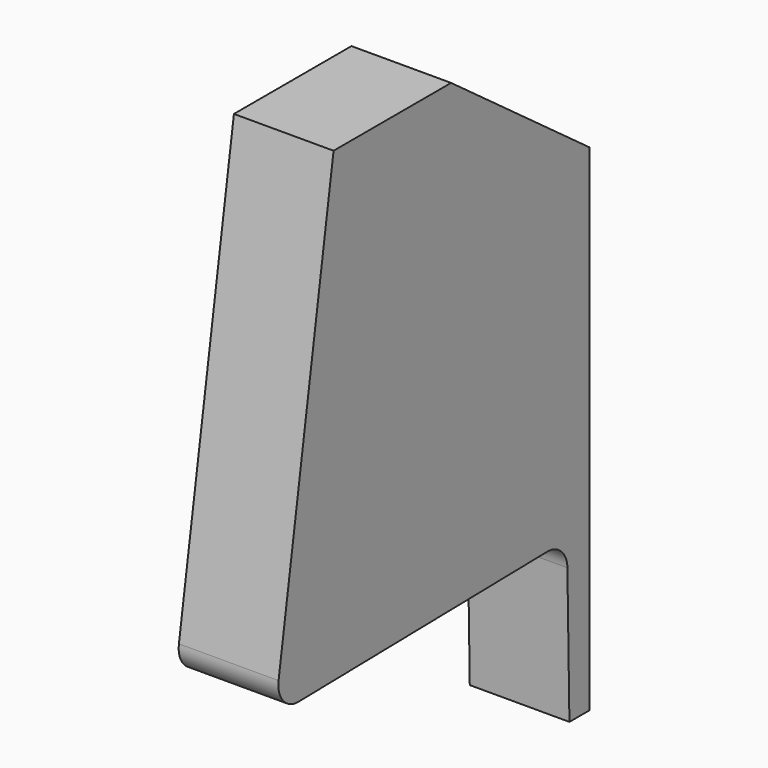
from build123d import *

# Parameters (mm, degrees)
F1_DEPTH = 25.4


# Not quite as in the source:
# - the program builds the solid bodies; features that only make, move or delete a surface that nothing else refers to are left out


with BuildPart() as f1:
    # F0 (on Right) → F1 (new body)
    with BuildSketch(Plane.YZ):
        with BuildLine():
            Line((30.5899139494, 31.8673923612), (-13.4478956461, 64.2119422555))
            Line((-13.4478956461, 64.2119422555), (-50.8971004581, 64.2119422555))
            Line((-50.8971004581, 64.2119422555), (-68.4238471531, -47.566784402))
            ThreePointArc((-68.4238471531, -47.566784402), (-66.9375558311, -52.7225543163), (-62.0332139244, -54.8993537478))
            Line((-62.0332139244, -54.8993537478), (17.1407288117, -53.4367848312))
            ThreePointArc((17.1407288117, -53.4367848312), (21.6644422357, -55.21340817), (23.6069282635, -59.6684190188))
            Line((23.6069282635, -59.6684190188), (24.2505592335, -94.5104021757))
            Line((24.2505592335, -94.5104021757), (30.5899139494, -94.5104021757))
            Line((30.5899139494, -94.5104021757), (30.5899139494, 31.8673923612))
        make_face()
    extrude(amount=F1_DEPTH)


solid = f1.part
